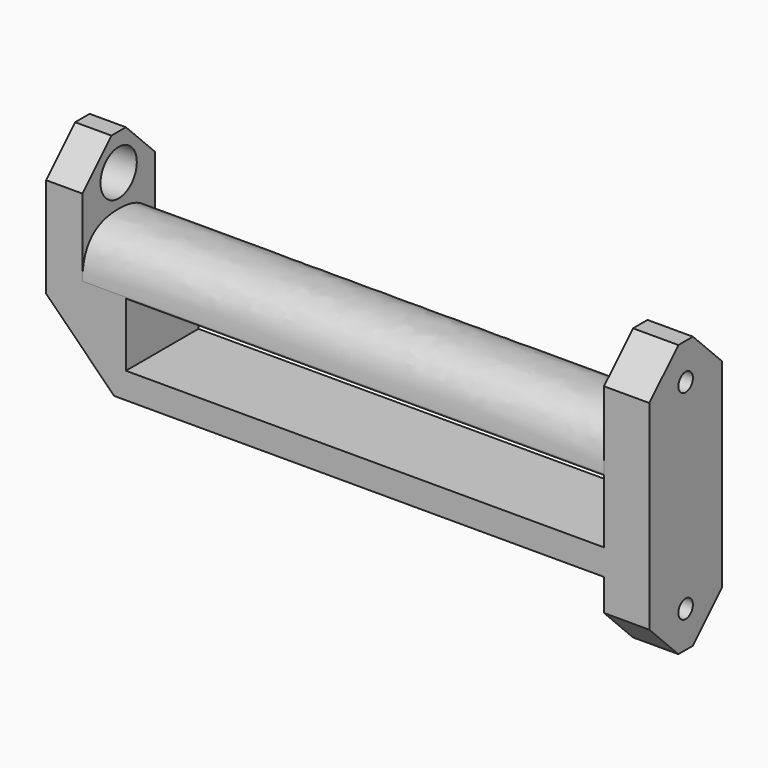
from build123d import *

# Parameters (mm, degrees)
F1_DEPTH       = 10
F2_T1_DEPTH    = 115
F3_SIZE        = 8
F5_D           = 4
F5_DEPTH       = 12
F5_CBORE_D     = 10
F5_CBORE_DEPTH = 5
F5_TIP         = 1.2017212381
F7_D           = 4
F7_DEPTH       = 12
F7_CBORE_D     = 10
F7_CBORE_DEPTH = 5
F7_TIP         = 1.2017212381
F8_SIZE        = 15
F9_R           = 5
F10_DEPTH      = 25


# Not quite as in the source:
# - a fillet or chamfer that OpenCascade refuses, or shapes differently, is made with other operations: its cross-section is extruded or revolved along the edge and cut away or added


with BuildPart() as f1:
    # F0 (on Front) → F1 (new body, symmetric)
    with BuildSketch(Plane.XZ):
        Polygon((57.5, 4.7522541136), (57.5, 15), (-57.5, 15), (-57.5, -15), (57.5, -15), (57.5, -9.264706634), (-47.9045920074, -9.264706634), (-47.9045920074, 4.7522541136), align=None)
        Polygon((57.5, 30), (57.5, 15), (57.5, 4.7522541136), (57.5, -9.264706634), (57.5, -15), (57.5, -30), (67.5, -30), (67.5, -15), (67.5, 15), (67.5, 30), align=None)
        Polygon((-57.5, -15), (-57.5, 15), (-57.5, 30), (-65.5, 30), (-65.5, -15), align=None)
    extrude(amount=F1_DEPTH, both=True)

    # F2: fillet of radius 10 on 2 edges, made by hand

    # F2_s2 → F2_t1 (cut)
    with BuildSketch(Plane.YZ.offset(-57.5)):
        with BuildLine():
            add(Edge.make_bspline(
                [(0, 15), (-10, 15), (-10, 5)],
                knots=[0, 0, 0, 1, 1, 1], degree=2, weights=[1, 1, 1]))
            Line((-10, 5), (-10.2, 5))
            Line((-10.2, 5), (-10.2, 15.2))
            Line((-10.2, 15.2), (0, 15.2))
            Line((0, 15.2), (0, 15))
        make_face()
        with BuildLine():
            add(Edge.make_bspline(
                [(0, 15), (10, 15), (10, 5)],
                knots=[0, 0, 0, 1, 1, 1], degree=2, weights=[1, 1, 1]))
            Line((10, 5), (10.2, 5))
            Line((10.2, 5), (10.2, 15.2))
            Line((10.2, 15.2), (0, 15.2))
            Line((0, 15.2), (0, 15))
        make_face()
    extrude(amount=F2_T1_DEPTH, mode=Mode.SUBTRACT)

    # F3
    f3_edges = [f1.edges().sort_by_distance(p)[0] for p in [
        (62.5, -10, -30),
        (62.5, 10, -30),
        (62.5, 10, 30),
        (62.5, -10, 30),
        (-61.5, -10, 30),
        (-61.5, 10, 30),
    ]]
    chamfer(f3_edges, length=F3_SIZE)

    # F5
    with Locations(Plane(origin=(57.5, 0, 0), x_dir=(0, -1, 0), z_dir=(-1, 0, 0))):
        with Locations((0, 22)):
            CounterBoreHole(F5_D / 2, F5_CBORE_D / 2, F5_CBORE_DEPTH, depth=F5_DEPTH)
            with Locations((0, 0, -(F5_DEPTH + F5_TIP / 2))):  # 118° drill point
                Cone(0, F5_D / 2, F5_TIP, mode=Mode.SUBTRACT)

    # F7
    with Locations(Plane(origin=(57.5, 0, 0), x_dir=(0, -1, 0), z_dir=(-1, 0, 0))):
        with Locations((0, -22)):
            CounterBoreHole(F7_D / 2, F7_CBORE_D / 2, F7_CBORE_DEPTH, depth=F7_DEPTH)
            with Locations((0, 0, -(F7_DEPTH + F7_TIP / 2))):  # 118° drill point
                Cone(0, F7_D / 2, F7_TIP, mode=Mode.SUBTRACT)

    # F8
    f8_edges = [f1.edges().sort_by_distance(p)[0] for p in [
        (-65.5, 0, -15),
    ]]
    chamfer(f8_edges, length=F8_SIZE)

    # F9 (on face) → F10 (cut)
    with BuildSketch(Plane.YZ.offset(-57.5)):
        with Locations((0, 22)):
            Circle(F9_R)
    extrude(amount=-F10_DEPTH, mode=Mode.SUBTRACT)


solid = f1.part
